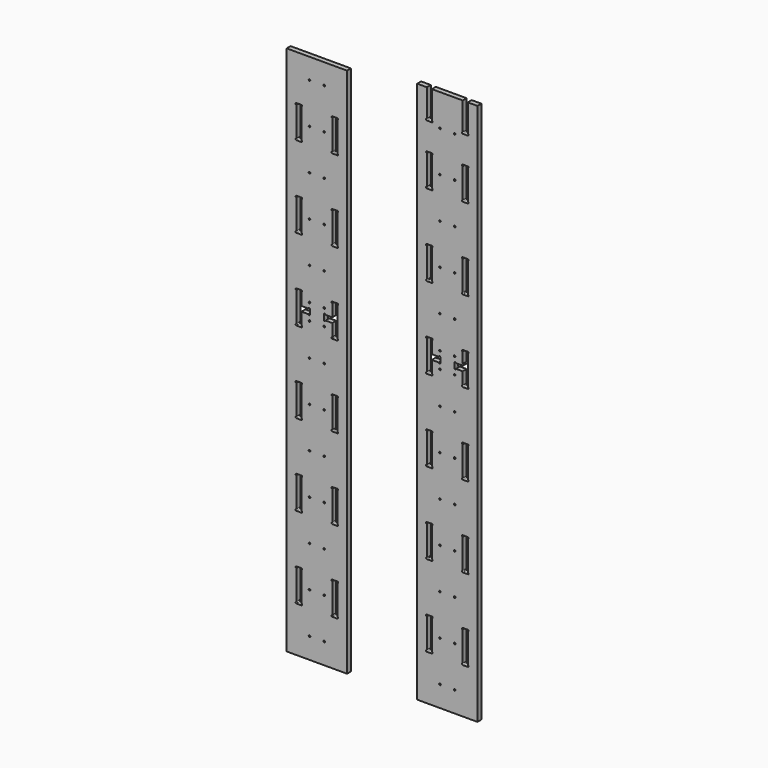
from build123d import *

# Parameters (mm, degrees)
F1_DEPTH = 18
F2_DEPTH = 18


# Not quite as in the source:
# - ends of sketch curves that miss each other by under 0.0002 mm in the source are joined


with BuildPart() as f1:
    # F0 (on Front) → F1 (new body)
    with BuildSketch(Plane.XZ):
        Polygon((-352.999778, -1175), (-352.999778, 777.505258), (-575.000001, 777.5052587556), (-575, -1175), align=None)
        with BuildLine():
            ThreePointArc((-491.003598, -1100.999773), (-493.1249183436, -1100.1210933436), (-494.003598, -1097.999773))
            ThreePointArc((-494.003598, -1097.999773), (-493.1249183436, -1095.8784526564), (-491.003598, -1094.999773))
            ThreePointArc((-491.003598, -1094.999773), (-488.8822776564, -1095.8784526564), (-488.003598, -1097.999773))
            ThreePointArc((-488.003598, -1097.999773), (-488.8822776564, -1100.1210933436), (-491.003598, -1100.999773))
        make_face(mode=Mode.SUBTRACT)
        with BuildLine():
            Line((-520.753598, -1008.249833), (-539.253616, -1008.249833))
            ThreePointArc((-539.253616, -1008.249833), (-542.263616, -1005.239833), (-539.253616, -1002.229833))
            Line((-539.253616, -1002.229833), (-539.253616, -893.769713))
            ThreePointArc((-539.253616, -893.769713), (-542.263616, -890.759713), (-539.253616, -887.749713))
            Line((-539.253616, -887.749713), (-520.753598, -887.749713))
            ThreePointArc((-520.753598, -887.749713), (-517.743598, -890.759713), (-520.753598, -893.769713))
            Line((-520.753598, -893.769713), (-520.753598, -1002.229833))
            ThreePointArc((-520.753598, -1002.229833), (-517.743598, -1005.239833), (-520.753598, -1008.249833))
        make_face(mode=Mode.SUBTRACT)
        with BuildLine():
            ThreePointArc((-491.003598, -950.999773), (-493.1249183436, -950.1210933436), (-494.003598, -947.999773))
            ThreePointArc((-494.003598, -947.999773), (-493.1249183436, -945.8784526564), (-491.003598, -944.999773))
            ThreePointArc((-491.003598, -944.999773), (-488.8822776564, -945.8784526564), (-488.003598, -947.999773))
            ThreePointArc((-488.003598, -947.999773), (-488.8822776564, -950.1210933436), (-491.003598, -950.999773))
        make_face(mode=Mode.SUBTRACT)
        with BuildLine():
            ThreePointArc((-437.003484, -1100.999773), (-439.1248043436, -1100.1210933436), (-440.003484, -1097.999773))
            ThreePointArc((-440.003484, -1097.999773), (-439.1248043436, -1095.8784526564), (-437.003484, -1094.999773))
            ThreePointArc((-437.003484, -1094.999773), (-434.8821636564, -1095.8784526564), (-434.003484, -1097.999773))
            ThreePointArc((-434.003484, -1097.999773), (-434.8821636564, -1100.1210933436), (-437.003484, -1100.999773))
        make_face(mode=Mode.SUBTRACT)
        with BuildLine():
            ThreePointArc((-437.003484, -950.999773), (-439.1248043436, -950.1210933436), (-440.003484, -947.999773))
            ThreePointArc((-440.003484, -947.999773), (-439.1248043436, -945.8784526564), (-437.003484, -944.999773))
            ThreePointArc((-437.003484, -944.999773), (-434.8821636564, -945.8784526564), (-434.003484, -947.999773))
            ThreePointArc((-434.003484, -947.999773), (-434.8821636564, -950.1210933436), (-437.003484, -950.999773))
        make_face(mode=Mode.SUBTRACT)
        with BuildLine():
            Line((-388.753466, -893.769713), (-388.753466, -1002.229833))
            ThreePointArc((-388.753466, -1002.229833), (-385.743466, -1005.239833), (-388.753466, -1008.249833))
            Line((-388.753466, -1008.249833), (-407.253484, -1008.249833))
            ThreePointArc((-407.253484, -1008.249833), (-410.263484, -1005.239833), (-407.253484, -1002.229833))
            Line((-407.253484, -1002.229833), (-407.253484, -893.769713))
            ThreePointArc((-407.253484, -893.769713), (-410.263484, -890.759713), (-407.253484, -887.749713))
            Line((-407.253484, -887.749713), (-388.753466, -887.749713))
            ThreePointArc((-388.753466, -887.749713), (-385.743466, -890.759713), (-388.753466, -893.769713))
        make_face(mode=Mode.SUBTRACT)
        with BuildLine():
            ThreePointArc((-491.003598, -800.999773), (-493.1249183436, -800.1210933436), (-494.003598, -797.999773))
            ThreePointArc((-494.003598, -797.999773), (-493.1249183436, -795.8784526564), (-491.003598, -794.999773))
            ThreePointArc((-491.003598, -794.999773), (-488.8822776564, -795.8784526564), (-488.003598, -797.999773))
            ThreePointArc((-488.003598, -797.999773), (-488.8822776564, -800.1210933436), (-491.003598, -800.999773))
        make_face(mode=Mode.SUBTRACT)
        with BuildLine():
            Line((-520.749918, -593.769409), (-520.749918, -702.229597))
            ThreePointArc((-520.749918, -702.229597), (-517.739918, -705.239597), (-520.749918, -708.249597))
            Line((-520.749918, -708.249597), (-539.249936, -708.249597))
            ThreePointArc((-539.249936, -708.249597), (-542.259936, -705.239597), (-539.249936, -702.229597))
            Line((-539.249936, -702.229597), (-539.249936, -593.769409))
            ThreePointArc((-539.249936, -593.769409), (-542.259936, -590.759409), (-539.249936, -587.749409))
            Line((-539.249936, -587.749409), (-520.749918, -587.749409))
            ThreePointArc((-520.749918, -587.749409), (-517.739918, -590.759409), (-520.749918, -593.769409))
        make_face(mode=Mode.SUBTRACT)
        with BuildLine():
            ThreePointArc((-491.003598, -650.999773), (-493.1249183436, -650.1210933436), (-494.003598, -647.999773))
            ThreePointArc((-494.003598, -647.999773), (-493.1249183436, -645.8784526564), (-491.003598, -644.999773))
            ThreePointArc((-491.003598, -644.999773), (-488.8822776564, -645.8784526564), (-488.003598, -647.999773))
            ThreePointArc((-488.003598, -647.999773), (-488.8822776564, -650.1210933436), (-491.003598, -650.999773))
        make_face(mode=Mode.SUBTRACT)
        with BuildLine():
            ThreePointArc((-437.003484, -800.999773), (-439.1248043436, -800.1210933436), (-440.003484, -797.999773))
            ThreePointArc((-440.003484, -797.999773), (-439.1248043436, -795.8784526564), (-437.003484, -794.999773))
            ThreePointArc((-437.003484, -794.999773), (-434.8821636564, -795.8784526564), (-434.003484, -797.999773))
            ThreePointArc((-434.003484, -797.999773), (-434.8821636564, -800.1210933436), (-437.003484, -800.999773))
        make_face(mode=Mode.SUBTRACT)
        with BuildLine():
            ThreePointArc((-437.003484, -650.999773), (-439.1248043436, -650.1210933436), (-440.003484, -647.999773))
            ThreePointArc((-440.003484, -647.999773), (-439.1248043436, -645.8784526564), (-437.003484, -644.999773))
            ThreePointArc((-437.003484, -644.999773), (-434.8821636564, -645.8784526564), (-434.003484, -647.999773))
            ThreePointArc((-434.003484, -647.999773), (-434.8821636564, -650.1210933436), (-437.003484, -650.999773))
        make_face(mode=Mode.SUBTRACT)
        with BuildLine():
            Line((-388.749807, -593.768176), (-388.749807, -702.228296))
            ThreePointArc((-388.749807, -702.228296), (-385.739807, -705.238296), (-388.749807, -708.248296))
            Line((-388.749807, -708.248296), (-407.249825, -708.248296))
            ThreePointArc((-407.249825, -708.248296), (-410.259825, -705.238296), (-407.249825, -702.228296))
            Line((-407.249825, -702.228296), (-407.249825, -593.768176))
            ThreePointArc((-407.249825, -593.768176), (-410.259825, -590.758176), (-407.249825, -587.748176))
            Line((-407.249825, -587.748176), (-388.749807, -587.748176))
            ThreePointArc((-388.749807, -587.748176), (-385.739807, -590.758176), (-388.749807, -593.768176))
        make_face(mode=Mode.SUBTRACT)
        with BuildLine():
            ThreePointArc((-491.003598, -500.999773), (-493.1249183436, -500.1210933436), (-494.003598, -497.999773))
            ThreePointArc((-494.003598, -497.999773), (-493.1249183436, -495.8784526564), (-491.003598, -494.999773))
            ThreePointArc((-491.003598, -494.999773), (-488.8822776564, -495.8784526564), (-488.003598, -497.999773))
            ThreePointArc((-488.003598, -497.999773), (-488.8822776564, -500.1210933436), (-491.003598, -500.999773))
        make_face(mode=Mode.SUBTRACT)
        with BuildLine():
            Line((-520.749849, -293.766172), (-520.749849, -402.226361))
            ThreePointArc((-520.749849, -402.226361), (-517.739849, -405.236361), (-520.749849, -408.246361))
            Line((-520.749849, -408.246361), (-539.249867, -408.246361))
            ThreePointArc((-539.249867, -408.246361), (-542.259867, -405.236361), (-539.249867, -402.226361))
            Line((-539.249867, -402.226361), (-539.249867, -293.766172))
            ThreePointArc((-539.249867, -293.766172), (-542.259867, -290.756172), (-539.249867, -287.746172))
            Line((-539.249867, -287.746172), (-520.749849, -287.746172))
            ThreePointArc((-520.749849, -287.746172), (-517.739849, -290.756172), (-520.749849, -293.766172))
        make_face(mode=Mode.SUBTRACT)
        with BuildLine():
            ThreePointArc((-491.003598, -350.999773), (-493.1249183436, -350.1210933436), (-494.003598, -347.999773))
            ThreePointArc((-494.003598, -347.999773), (-493.1249183436, -345.8784526564), (-491.003598, -344.999773))
            ThreePointArc((-491.003598, -344.999773), (-488.8822776564, -345.8784526564), (-488.003598, -347.999773))
            ThreePointArc((-488.003598, -347.999773), (-488.8822776564, -350.1210933436), (-491.003598, -350.999773))
        make_face(mode=Mode.SUBTRACT)
        with BuildLine():
            ThreePointArc((-437.003484, -500.999773), (-439.1248043436, -500.1210933436), (-440.003484, -497.999773))
            ThreePointArc((-440.003484, -497.999773), (-439.1248043436, -495.8784526564), (-437.003484, -494.999773))
            ThreePointArc((-437.003484, -494.999773), (-434.8821636564, -495.8784526564), (-434.003484, -497.999773))
            ThreePointArc((-434.003484, -497.999773), (-434.8821636564, -500.1210933436), (-437.003484, -500.999773))
        make_face(mode=Mode.SUBTRACT)
        with BuildLine():
            ThreePointArc((-437.003484, -350.999773), (-439.1248043436, -350.1210933436), (-440.003484, -347.999773))
            ThreePointArc((-440.003484, -347.999773), (-439.1248043436, -345.8784526564), (-437.003484, -344.999773))
            ThreePointArc((-437.003484, -344.999773), (-434.8821636564, -345.8784526564), (-434.003484, -347.999773))
            ThreePointArc((-434.003484, -347.999773), (-434.8821636564, -350.1210933436), (-437.003484, -350.999773))
        make_face(mode=Mode.SUBTRACT)
        with BuildLine():
            Line((-407.249756, -402.225059), (-407.249756, -293.764939))
            ThreePointArc((-407.249756, -293.764939), (-410.259756, -290.754939), (-407.249756, -287.744939))
            Line((-407.249756, -287.744939), (-388.749738, -287.744939))
            ThreePointArc((-388.749738, -287.744939), (-385.739738, -290.754939), (-388.749738, -293.764939))
            Line((-388.749738, -293.764939), (-388.749738, -402.225059))
            ThreePointArc((-388.749738, -402.225059), (-385.739738, -405.235059), (-388.749738, -408.245059))
            Line((-388.749738, -408.245059), (-407.249756, -408.245059))
            ThreePointArc((-407.249756, -408.245059), (-410.259756, -405.235059), (-407.249756, -402.225059))
        make_face(mode=Mode.SUBTRACT)
        with BuildLine():
            ThreePointArc((-491.003598, -200.999773), (-493.1249183436, -200.1210933436), (-494.003598, -197.999773))
            ThreePointArc((-494.003598, -197.999773), (-493.1249183436, -195.8784526564), (-491.003598, -194.999773))
            ThreePointArc((-491.003598, -194.999773), (-488.8822776564, -195.8784526564), (-488.003598, -197.999773))
            ThreePointArc((-488.003598, -197.999773), (-488.8822776564, -200.1210933436), (-491.003598, -200.999773))
        make_face(mode=Mode.SUBTRACT)
        with BuildLine():
            ThreePointArc((-491.003598, -80.986601), (-493.1249183436, -80.1079213436), (-494.003598, -77.986601))
            ThreePointArc((-494.003598, -77.986601), (-493.1249183436, -75.8652806564), (-491.003598, -74.986601))
            ThreePointArc((-491.003598, -74.986601), (-488.8822776564, -75.8652806564), (-488.003598, -77.986601))
            ThreePointArc((-488.003598, -77.986601), (-488.8822776564, -80.1079213436), (-491.003598, -80.986601))
        make_face(mode=Mode.SUBTRACT)
        with BuildLine():
            Line((-520.749955, 6.236645), (-520.749974, -38.743178))
            Line((-520.749974, -38.743178), (-495.769943, -38.743178))
            ThreePointArc((-495.769943, -38.743178), (-492.759943, -35.733178), (-489.749943, -38.743178))
            Line((-489.749943, -38.743178), (-489.749943, -57.243196))
            ThreePointArc((-489.749943, -57.243196), (-492.759943, -60.253196), (-495.769943, -57.243196))
            Line((-495.769943, -57.243196), (-520.749974, -57.243196))
            Line((-520.749974, -57.243196), (-520.749955, -102.223475))
            ThreePointArc((-520.749955, -102.223475), (-517.739954, -105.233474), (-520.749953, -108.243475))
            Line((-520.749953, -108.243475), (-539.249971, -108.243475))
            ThreePointArc((-539.249971, -108.243475), (-542.259971, -105.233475), (-539.249971, -102.223475))
            Line((-539.249971, -102.223475), (-539.249971, 6.236645))
            ThreePointArc((-539.249971, 6.236645), (-542.259971, 9.246645), (-539.249971, 12.256645))
            Line((-539.249971, 12.256645), (-520.749953, 12.256645))
            ThreePointArc((-520.749953, 12.256645), (-517.739954, 9.246644), (-520.749955, 6.236645))
        make_face(mode=Mode.SUBTRACT)
        with BuildLine():
            ThreePointArc((-491.003598, -20.999773), (-493.1249183436, -20.1210933436), (-494.003598, -17.999773))
            ThreePointArc((-494.003598, -17.999773), (-493.1249183436, -15.8784526564), (-491.003598, -14.999773))
            ThreePointArc((-491.003598, -14.999773), (-488.8822776564, -15.8784526564), (-488.003598, -17.999773))
            ThreePointArc((-488.003598, -17.999773), (-488.8822776564, -20.1210933436), (-491.003598, -20.999773))
        make_face(mode=Mode.SUBTRACT)
        with BuildLine():
            ThreePointArc((-437.003484, -200.999773), (-439.1248043436, -200.1210933436), (-440.003484, -197.999773))
            ThreePointArc((-440.003484, -197.999773), (-439.1248043436, -195.8784526564), (-437.003484, -194.999773))
            ThreePointArc((-437.003484, -194.999773), (-434.8821636564, -195.8784526564), (-434.003484, -197.999773))
            ThreePointArc((-434.003484, -197.999773), (-434.8821636564, -200.1210933436), (-437.003484, -200.999773))
        make_face(mode=Mode.SUBTRACT)
        with BuildLine():
            ThreePointArc((-437.003484, -80.986601), (-439.1248043436, -80.1079213436), (-440.003484, -77.986601))
            ThreePointArc((-440.003484, -77.986601), (-439.1248043436, -75.8652806564), (-437.003484, -74.986601))
            ThreePointArc((-437.003484, -74.986601), (-434.8821636564, -75.8652806564), (-434.003484, -77.986601))
            ThreePointArc((-434.003484, -77.986601), (-434.8821636564, -80.1079213436), (-437.003484, -80.986601))
        make_face(mode=Mode.SUBTRACT)
        with BuildLine():
            ThreePointArc((-437.003484, -20.999773), (-439.1248043436, -20.1210933436), (-440.003484, -17.999773))
            ThreePointArc((-440.003484, -17.999773), (-439.1248043436, -15.8784526564), (-437.003484, -14.999773))
            ThreePointArc((-437.003484, -14.999773), (-434.8821636564, -15.8784526564), (-434.003484, -17.999773))
            ThreePointArc((-434.003484, -17.999773), (-434.8821636564, -20.1210933436), (-437.003484, -20.999773))
        make_face(mode=Mode.SUBTRACT)
        with BuildLine():
            Line((-388.749842, 6.235389), (-388.749842, -102.224782))
            ThreePointArc((-388.749842, -102.224782), (-385.739842, -105.234782), (-388.749842, -108.244782))
            Line((-388.749842, -108.244782), (-407.249855, -108.244782))
            ThreePointArc((-407.249855, -108.2447819994), (-410.2599159994, -105.2348425), (-407.249976, -102.2247820006))
            Line((-407.249976, -102.224782), (-407.250887, -57.243196))
            Line((-407.250887, -57.243196), (-432.230923, -57.243196))
            ThreePointArc((-432.230923, -57.243196), (-435.240923, -60.253196), (-438.250923, -57.243196))
            Line((-438.250923, -57.243196), (-438.250923, -38.743178))
            ThreePointArc((-438.250923, -38.743178), (-435.240923, -35.733178), (-432.230923, -38.743178))
            Line((-432.230923, -38.743178), (-407.250887, -38.743178))
            Line((-407.250887, -38.743178), (-407.249976, 6.235389))
            ThreePointArc((-407.249976, 6.2353890006), (-410.2599159994, 9.2454495), (-407.249855, 12.2553889994))
            Line((-407.249855, 12.255389), (-388.749842, 12.255389))
            ThreePointArc((-388.749842, 12.255389), (-385.739842, 9.245389), (-388.749842, 6.235389))
        make_face(mode=Mode.SUBTRACT)
        with BuildLine():
            ThreePointArc((-491.003598, 99.000227), (-493.1249183436, 99.8789066564), (-494.003598, 102.000227))
            ThreePointArc((-494.003598, 102.000227), (-493.1249183436, 104.1215473436), (-491.003598, 105.000227))
            ThreePointArc((-491.003598, 105.000227), (-488.8822776564, 104.1215473436), (-488.003598, 102.000227))
            ThreePointArc((-488.003598, 102.000227), (-488.8822776564, 99.8789066564), (-491.003598, 99.000227))
        make_face(mode=Mode.SUBTRACT)
        with BuildLine():
            Line((-520.749918, 306.234452), (-520.749918, 197.774263))
            ThreePointArc((-520.749918, 197.774263), (-517.739918, 194.764263), (-520.749918, 191.754263))
            Line((-520.749918, 191.754263), (-539.249936, 191.754263))
            ThreePointArc((-539.249936, 191.754263), (-542.259936, 194.764263), (-539.249936, 197.774263))
            Line((-539.249936, 197.774263), (-539.249936, 306.234452))
            ThreePointArc((-539.249936, 306.234452), (-542.259936, 309.244452), (-539.249936, 312.254452))
            Line((-539.249936, 312.254452), (-520.749918, 312.254452))
            ThreePointArc((-520.749918, 312.254452), (-517.739918, 309.244452), (-520.749918, 306.234452))
        make_face(mode=Mode.SUBTRACT)
        with BuildLine():
            ThreePointArc((-491.003598, 249.000227), (-493.1249183436, 249.8789066564), (-494.003598, 252.000227))
            ThreePointArc((-494.003598, 252.000227), (-493.1249183436, 254.1215473436), (-491.003598, 255.000227))
            ThreePointArc((-491.003598, 255.000227), (-488.8822776564, 254.1215473436), (-488.003598, 252.000227))
            ThreePointArc((-488.003598, 252.000227), (-488.8822776564, 249.8789066564), (-491.003598, 249.000227))
        make_face(mode=Mode.SUBTRACT)
        with BuildLine():
            ThreePointArc((-437.003484, 99.000227), (-439.1248043436, 99.8789066564), (-440.003484, 102.000227))
            ThreePointArc((-440.003484, 102.000227), (-439.1248043436, 104.1215473436), (-437.003484, 105.000227))
            ThreePointArc((-437.003484, 105.000227), (-434.8821636564, 104.1215473436), (-434.003484, 102.000227))
            ThreePointArc((-434.003484, 102.000227), (-434.8821636564, 99.8789066564), (-437.003484, 99.000227))
        make_face(mode=Mode.SUBTRACT)
        with BuildLine():
            ThreePointArc((-437.003484, 249.000227), (-439.1248043436, 249.8789066564), (-440.003484, 252.000227))
            ThreePointArc((-440.003484, 252.000227), (-439.1248043436, 254.1215473436), (-437.003484, 255.000227))
            ThreePointArc((-437.003484, 255.000227), (-434.8821636564, 254.1215473436), (-434.003484, 252.000227))
            ThreePointArc((-434.003484, 252.000227), (-434.8821636564, 249.8789066564), (-437.003484, 249.000227))
        make_face(mode=Mode.SUBTRACT)
        with BuildLine():
            Line((-407.249825, 197.775565), (-407.249825, 306.235685))
            ThreePointArc((-407.249825, 306.235685), (-410.259825, 309.245685), (-407.249825, 312.255685))
            Line((-407.249825, 312.255685), (-388.749807, 312.255685))
            ThreePointArc((-388.749807, 312.255685), (-385.739807, 309.245685), (-388.749807, 306.235685))
            Line((-388.749807, 306.235685), (-388.749807, 197.775565))
            ThreePointArc((-388.749807, 197.775565), (-385.739807, 194.765565), (-388.749807, 191.755565))
            Line((-388.749807, 191.755565), (-407.249825, 191.755565))
            ThreePointArc((-407.249825, 191.755565), (-410.259825, 194.765565), (-407.249825, 197.775565))
        make_face(mode=Mode.SUBTRACT)
        with BuildLine():
            ThreePointArc((-491.003598, 399.000227), (-493.1249183436, 399.8789066564), (-494.003598, 402.000227))
            ThreePointArc((-494.003598, 402.000227), (-493.1249183436, 404.1215473436), (-491.003598, 405.000227))
            ThreePointArc((-491.003598, 405.000227), (-488.8822776564, 404.1215473436), (-488.003598, 402.000227))
            ThreePointArc((-488.003598, 402.000227), (-488.8822776564, 399.8789066564), (-491.003598, 399.000227))
        make_face(mode=Mode.SUBTRACT)
        with BuildLine():
            Line((-539.249936, 497.774554), (-539.249936, 606.234743))
            ThreePointArc((-539.249936, 606.234743), (-542.259936, 609.244743), (-539.249936, 612.254743))
            Line((-539.249936, 612.254743), (-520.749918, 612.254743))
            ThreePointArc((-520.749918, 612.254743), (-517.739918, 609.244743), (-520.749918, 606.234743))
            Line((-520.749918, 606.234743), (-520.749918, 497.774554))
            ThreePointArc((-520.749918, 497.774554), (-517.739918, 494.764554), (-520.749918, 491.754554))
            Line((-520.749918, 491.754554), (-539.249936, 491.754554))
            ThreePointArc((-539.249936, 491.754554), (-542.259936, 494.764554), (-539.249936, 497.774554))
        make_face(mode=Mode.SUBTRACT)
        with BuildLine():
            ThreePointArc((-491.003598, 549.000227), (-493.1249183436, 549.8789066564), (-494.003598, 552.000227))
            ThreePointArc((-494.003598, 552.000227), (-493.1249183436, 554.1215473436), (-491.003598, 555.000227))
            ThreePointArc((-491.003598, 555.000227), (-488.8822776564, 554.1215473436), (-488.003598, 552.000227))
            ThreePointArc((-488.003598, 552.000227), (-488.8822776564, 549.8789066564), (-491.003598, 549.000227))
        make_face(mode=Mode.SUBTRACT)
        with BuildLine():
            ThreePointArc((-437.003484, 399.000227), (-439.1248043436, 399.8789066564), (-440.003484, 402.000227))
            ThreePointArc((-440.003484, 402.000227), (-439.1248043436, 404.1215473436), (-437.003484, 405.000227))
            ThreePointArc((-437.003484, 405.000227), (-434.8821636564, 404.1215473436), (-434.003484, 402.000227))
            ThreePointArc((-434.003484, 402.000227), (-434.8821636564, 399.8789066564), (-437.003484, 399.000227))
        make_face(mode=Mode.SUBTRACT)
        with BuildLine():
            ThreePointArc((-437.003484, 549.000227), (-439.1248043436, 549.8789066564), (-440.003484, 552.000227))
            ThreePointArc((-440.003484, 552.000227), (-439.1248043436, 554.1215473436), (-437.003484, 555.000227))
            ThreePointArc((-437.003484, 555.000227), (-434.8821636564, 554.1215473436), (-434.003484, 552.000227))
            ThreePointArc((-434.003484, 552.000227), (-434.8821636564, 549.8789066564), (-437.003484, 549.000227))
        make_face(mode=Mode.SUBTRACT)
        with BuildLine():
            Line((-388.749807, 606.235976), (-388.749807, 497.775856))
            ThreePointArc((-388.749807, 497.775856), (-385.739807, 494.765856), (-388.749807, 491.755856))
            Line((-388.749807, 491.755856), (-407.249825, 491.755856))
            ThreePointArc((-407.249825, 491.755856), (-410.259825, 494.765856), (-407.249825, 497.775856))
            Line((-407.249825, 497.775856), (-407.249825, 606.235976))
            ThreePointArc((-407.249825, 606.235976), (-410.259825, 609.245976), (-407.249825, 612.255976))
            Line((-407.249825, 612.255976), (-388.749807, 612.255976))
            ThreePointArc((-388.749807, 612.255976), (-385.739807, 609.245976), (-388.749807, 606.235976))
        make_face(mode=Mode.SUBTRACT)
        Polygon((-506.973918, 655.086016), (-522.336584, 655.086016), (-522.336584, 672.56035), (-506.973918, 672.56035), (-506.541339, 672.557371), (-506.111272, 672.53204), (-505.684535, 672.484696), (-505.261944, 672.415683), (-504.844315, 672.325341), (-504.432466, 672.214014), (-504.027214, 672.082041), (-503.629376, 671.929766), (-503.239768, 671.75753), (-502.859207, 671.565675), (-502.488511, 671.354543), (-502.128496, 671.124475), (-501.779978, 670.875813), (-501.443776, 670.608899), (-501.120706, 670.324075), (-500.811584, 670.021683), (-500.5137, 669.714114), (-500.232763, 669.39305), (-499.969092, 669.059272), (-499.723011, 668.713558), (-499.49484, 668.356688), (-499.284901, 667.989441), (-499.093514, 667.612596), (-498.921001, 667.226933), (-498.767683, 666.833231), (-498.633882, 666.432269), (-498.519919, 666.024827), (-498.426115, 665.611683), (-498.352792, 665.193618), (-498.30027, 664.77141), (-498.268872, 664.345838), (-498.258918, 663.917683), (-498.256319, 663.478817), (-498.276304, 663.042145), (-498.318539, 662.608495), (-498.382694, 662.178693), (-498.468436, 661.753568), (-498.575435, 661.333945), (-498.703359, 660.920652), (-498.851876, 660.514516), (-499.020655, 660.116365), (-499.209363, 659.727025), (-499.417671, 659.347324), (-499.645246, 658.978089), (-499.891756, 658.620147), (-500.15687, 658.274325), (-500.440257, 657.94145), (-500.741584, 657.62235), (-501.056696, 657.32124), (-501.385493, 657.037626), (-501.727169, 656.771834), (-502.080918, 656.524188), (-502.445932, 656.295013), (-502.821404, 656.084633), (-503.20653, 655.893373), (-503.600501, 655.721558), (-504.002511, 655.569512), (-504.411753, 655.437561), (-504.827422, 655.326029), (-505.248709, 655.23524), (-505.674809, 655.16552), (-506.104915, 655.117193), (-506.53822, 655.090583), align=None, mode=Mode.SUBTRACT)
        Polygon((-475.769852, 637.107772), (-476.131918, 637.10535), (-476.499301, 637.102372), (-476.8659, 637.108707), (-477.231546, 637.124288), (-477.596071, 637.14905), (-477.959305, 637.182925), (-478.32108, 637.225848), (-478.681228, 637.277753), (-479.039579, 637.338574), (-479.395965, 637.408243), (-479.750216, 637.486695), (-480.102165, 637.573864), (-480.451642, 637.669684), (-480.798479, 637.774087), (-481.142506, 637.887009), (-481.483556, 638.008382), (-481.821459, 638.138141), (-482.156047, 638.27622), (-482.48715, 638.422551), (-482.814601, 638.577069), (-483.138229, 638.739708), (-483.457868, 638.910402), (-483.773347, 639.089083), (-484.084498, 639.275687), (-484.391152, 639.470147), (-484.693141, 639.672395), (-484.990295, 639.882368), (-485.282446, 640.099997), (-485.569426, 640.325217), (-485.851065, 640.557962), (-486.127195, 640.798166), (-486.397646, 641.045761), (-486.662251, 641.300683), (-486.968379, 641.633429), (-487.26546, 641.973094), (-487.553417, 642.319472), (-487.832171, 642.672359), (-488.101646, 643.031551), (-488.361764, 643.396843), (-488.612446, 643.76803), (-488.853615, 644.144907), (-489.085194, 644.52727), (-489.307104, 644.914914), (-489.519267, 645.307635), (-489.721606, 645.705228), (-489.914044, 646.107488), (-490.096502, 646.51421), (-490.268902, 646.925191), (-490.431168, 647.340225), (-490.58322, 647.759107), (-490.724982, 648.181633), (-490.856375, 648.607599), (-490.977322, 649.0368), (-491.087746, 649.46903), (-491.187567, 649.904086), (-491.27671, 650.341762), (-491.355095, 650.781855), (-491.422645, 651.224159), (-491.479282, 651.66847), (-491.524929, 652.114583), (-491.559507, 652.562293), (-491.58294, 653.011396), (-491.595149, 653.461688), (-491.596056, 653.912963), (-491.585584, 654.365016), (-491.599646, 654.855997), (-491.601202, 655.346163), (-491.590337, 655.835287), (-491.567136, 656.323143), (-491.531686, 656.809504), (-491.484071, 657.294142), (-491.424376, 657.776831), (-491.352688, 658.257344), (-491.269092, 658.735455), (-491.173673, 659.210935), (-491.066517, 659.68356), (-490.947709, 660.1531), (-490.817335, 660.619331), (-490.675479, 661.082024), (-490.522228, 661.540953), (-490.357668, 661.995891), (-490.181882, 662.446612), (-489.994957, 662.892888), (-489.796979, 663.334492), (-489.588032, 663.771198), (-489.368203, 664.202779), (-489.137576, 664.629007), (-488.896237, 665.049657), (-488.644272, 665.464501), (-488.381765, 665.873312), (-488.108804, 666.275863), (-487.825472, 666.671928), (-487.531855, 667.06128), (-487.228039, 667.443692), (-486.91411, 667.818936), (-486.590152, 668.186787), (-486.256251, 668.547016), (-486.006221, 668.801356), (-485.750182, 669.048515), (-485.488307, 669.288422), (-485.220766, 669.521005), (-484.94773, 669.746194), (-484.669372, 669.963916), (-484.385861, 670.174102), (-484.097371, 670.376678), (-483.804071, 670.571574), (-483.506133, 670.758718), (-483.203729, 670.93804), (-482.89703, 671.109467), (-482.586207, 671.272929), (-482.271432, 671.428354), (-481.952875, 671.575671), (-481.630709, 671.714808), (-481.305104, 671.845694), (-480.976233, 671.968258), (-480.644265, 672.082428), (-480.309373, 672.188133), (-479.971727, 672.285301), (-479.6315, 672.373862), (-479.288862, 672.453744), (-478.943985, 672.524876), (-478.59704, 672.587185), (-478.248199, 672.640602), (-477.897632, 672.685054), (-477.545512, 672.72047), (-477.192009, 672.746779), (-476.837295, 672.76391), (-476.48154, 672.77179), (-476.124918, 672.77035), (-475.76245, 672.767135), (-475.400977, 672.754479), (-475.040671, 672.732456), (-474.681705, 672.701138), (-474.324254, 672.6606), (-473.96849, 672.610917), (-473.614588, 672.552161), (-473.26272, 672.484407), (-472.91306, 672.407729), (-472.565781, 672.3222), (-472.221057, 672.227895), (-471.879062, 672.124887), (-471.539969, 672.01325), (-471.203951, 671.893059), (-470.871181, 671.764387), (-470.541834, 671.627308), (-470.216083, 671.481896), (-469.894101, 671.328225), (-469.576061, 671.166369), (-469.262138, 670.996401), (-468.952504, 670.818396), (-468.647333, 670.632428), (-468.346798, 670.43857), (-468.051074, 670.236897), (-467.760333, 670.027481), (-467.474748, 669.810398), (-467.194494, 669.585722), (-466.919744, 669.353525), (-466.650671, 669.113882), (-466.387449, 668.866867), (-466.130251, 668.612554), (-465.879251, 668.351016), (-465.555343, 667.992679), (-465.241237, 667.627003), (-464.937012, 667.25421), (-464.642748, 666.874522), (-464.358527, 666.48816), (-464.084428, 666.095347), (-463.820531, 665.696303), (-463.566918, 665.291251), (-463.323667, 664.880412), (-463.090861, 664.464008), (-462.868578, 664.042261), (-462.656899, 663.615393), (-462.455905, 663.183625), (-462.265676, 662.74718), (-462.086292, 662.306278), (-461.917834, 661.861141), (-461.760382, 661.411992), (-461.614015, 660.959052), (-461.478816, 660.502543), (-461.354863, 660.042686), (-461.242237, 659.579704), (-461.141019, 659.113817), (-461.051288, 658.645249), (-460.973126, 658.174219), (-460.906612, 657.700951), (-460.851827, 657.225666), (-460.808851, 656.748586), (-460.777764, 656.269932), (-460.758647, 655.789927), (-460.75158, 655.308791), (-460.756643, 654.826747), (-460.773918, 654.344016), (-460.766542, 653.893542), (-460.770611, 653.443945), (-460.786045, 652.995432), (-460.812764, 652.548211), (-460.850687, 652.102489), (-460.899733, 651.658472), (-460.959823, 651.216369), (-461.030876, 650.776386), (-461.112812, 650.338731), (-461.20555, 649.903611), (-461.30901, 649.471232), (-461.423113, 649.041803), (-461.547777, 648.615531), (-461.682922, 648.192622), (-461.828468, 647.773284), (-461.984334, 647.357725), (-462.150441, 646.94615), (-462.326708, 646.538768), (-462.513054, 646.135786), (-462.709399, 645.737411), (-462.915664, 645.343851), (-463.131767, 644.955311), (-463.357628, 644.572001), (-463.593168, 644.194126), (-463.838305, 643.821894), (-464.092959, 643.455512), (-464.35705, 643.095188), (-464.630498, 642.741129), (-464.913223, 642.393542), (-465.205143, 642.052633), (-465.506179, 641.718611), (-465.816251, 641.391683), (-466.073419, 641.136871), (-466.336438, 640.889169), (-466.605143, 640.648646), (-466.879371, 640.41537), (-467.158957, 640.18941), (-467.443735, 639.970835), (-467.733543, 639.759714), (-468.028214, 639.556115), (-468.327586, 639.360108), (-468.631492, 639.171761), (-468.939769, 638.991142), (-469.252253, 638.818322), (-469.568778, 638.653367), (-469.88918, 638.496348), (-470.213296, 638.347333), (-470.540959, 638.206391), (-470.872006, 638.073591), (-471.206273, 637.949001), (-471.543594, 637.83269), (-471.883806, 637.724727), (-472.226744, 637.62518), (-472.572243, 637.53412), (-472.920138, 637.451613), (-473.270266, 637.37773), (-473.622462, 637.312538), (-473.976562, 637.256108), (-474.3324, 637.208506), (-474.689813, 637.169803), (-475.048635, 637.140067), (-475.408703, 637.119367), align=None, mode=Mode.SUBTRACT)
        with BuildLine():
            ThreePointArc((-491.003598, 699.000227), (-493.1249183436, 699.8789066564), (-494.003598, 702.000227))
            ThreePointArc((-494.003598, 702.000227), (-493.1249183436, 704.1215473436), (-491.003598, 705.000227))
            ThreePointArc((-491.003598, 705.000227), (-488.8822776564, 704.1215473436), (-488.003598, 702.000227))
            ThreePointArc((-488.003598, 702.000227), (-488.8822776564, 699.8789066564), (-491.003598, 699.000227))
        make_face(mode=Mode.SUBTRACT)
        Polygon((-437.055185, 637.107772), (-437.417251, 637.10535), (-437.784634, 637.102372), (-438.151233, 637.108707), (-438.516879, 637.124288), (-438.881404, 637.14905), (-439.244638, 637.182925), (-439.606414, 637.225848), (-439.966561, 637.277753), (-440.324912, 637.338574), (-440.681298, 637.408243), (-441.03555, 637.486695), (-441.387498, 637.573864), (-441.736975, 637.669684), (-442.083812, 637.774087), (-442.42784, 637.887009), (-442.768889, 638.008382), (-443.106793, 638.138141), (-443.44138, 638.27622), (-443.772484, 638.422551), (-444.099934, 638.577069), (-444.423563, 638.739708), (-444.743201, 638.910402), (-445.05868, 639.089083), (-445.369831, 639.275687), (-445.676485, 639.470147), (-445.978474, 639.672395), (-446.275628, 639.882368), (-446.56778, 640.099997), (-446.854759, 640.325217), (-447.136398, 640.557962), (-447.412528, 640.798166), (-447.682979, 641.045761), (-447.947584, 641.300683), (-448.253712, 641.633429), (-448.550793, 641.973094), (-448.83875, 642.319472), (-449.117505, 642.672359), (-449.38698, 643.031551), (-449.647097, 643.396843), (-449.89778, 643.76803), (-450.138949, 644.144907), (-450.370527, 644.52727), (-450.592437, 644.914914), (-450.8046, 645.307635), (-451.00694, 645.705228), (-451.199377, 646.107488), (-451.381835, 646.51421), (-451.554235, 646.925191), (-451.716501, 647.340225), (-451.868553, 647.759107), (-452.010315, 648.181633), (-452.141709, 648.607599), (-452.262656, 649.0368), (-452.373079, 649.46903), (-452.472901, 649.904086), (-452.562043, 650.341762), (-452.640428, 650.781855), (-452.707978, 651.224159), (-452.764615, 651.66847), (-452.810262, 652.114583), (-452.844841, 652.562293), (-452.868273, 653.011396), (-452.880482, 653.461688), (-452.881389, 653.912963), (-452.870918, 654.365016), (-452.88498, 654.855997), (-452.886535, 655.346163), (-452.87567, 655.835287), (-452.85247, 656.323143), (-452.817019, 656.809504), (-452.769404, 657.294142), (-452.70971, 657.776831), (-452.638022, 658.257344), (-452.554426, 658.735455), (-452.459007, 659.210935), (-452.351851, 659.68356), (-452.233043, 660.1531), (-452.102668, 660.619331), (-451.960813, 661.082024), (-451.807562, 661.540953), (-451.643001, 661.995891), (-451.467215, 662.446612), (-451.280291, 662.892888), (-451.082312, 663.334492), (-450.873365, 663.771198), (-450.653536, 664.202779), (-450.422909, 664.629007), (-450.18157, 665.049657), (-449.929605, 665.464501), (-449.667099, 665.873312), (-449.394137, 666.275863), (-449.110805, 666.671928), (-448.817188, 667.06128), (-448.513373, 667.443692), (-448.199443, 667.818936), (-447.875485, 668.186787), (-447.541584, 668.547016), (-447.291554, 668.801356), (-447.035516, 669.048515), (-446.77364, 669.288422), (-446.506099, 669.521005), (-446.233064, 669.746194), (-445.954705, 669.963916), (-445.671195, 670.174102), (-445.382704, 670.376678), (-445.089404, 670.571574), (-444.791467, 670.758718), (-444.489063, 670.93804), (-444.182363, 671.109467), (-443.871541, 671.272929), (-443.556765, 671.428354), (-443.238209, 671.575671), (-442.916043, 671.714808), (-442.590438, 671.845694), (-442.261566, 671.968258), (-441.929598, 672.082428), (-441.594706, 672.188133), (-441.257061, 672.285301), (-440.916833, 672.373862), (-440.574196, 672.453744), (-440.229319, 672.524876), (-439.882374, 672.587185), (-439.533532, 672.640602), (-439.182966, 672.685054), (-438.830845, 672.72047), (-438.477342, 672.746779), (-438.122628, 672.76391), (-437.766874, 672.77179), (-437.410251, 672.77035), (-437.047784, 672.767135), (-436.68631, 672.754479), (-436.326004, 672.732456), (-435.967039, 672.701138), (-435.609587, 672.6606), (-435.253824, 672.610917), (-434.899921, 672.552161), (-434.548053, 672.484407), (-434.198393, 672.407729), (-433.851114, 672.3222), (-433.506391, 672.227895), (-433.164395, 672.124887), (-432.825302, 672.01325), (-432.489284, 671.893059), (-432.156515, 671.764387), (-431.827168, 671.627308), (-431.501416, 671.481896), (-431.179434, 671.328225), (-430.861394, 671.166369), (-430.547471, 670.996401), (-430.237837, 670.818396), (-429.932666, 670.632428), (-429.632132, 670.43857), (-429.336407, 670.236897), (-429.045666, 670.027481), (-428.760082, 669.810398), (-428.479828, 669.585722), (-428.205078, 669.353525), (-427.936005, 669.113882), (-427.672783, 668.866867), (-427.415585, 668.612554), (-427.164584, 668.351016), (-426.840677, 667.992679), (-426.52657, 667.627003), (-426.222345, 667.25421), (-425.928082, 666.874522), (-425.64386, 666.48816), (-425.369761, 666.095347), (-425.105864, 665.696303), (-424.852251, 665.291251), (-424.609001, 664.880412), (-424.376194, 664.464008), (-424.153911, 664.042261), (-423.942233, 663.615393), (-423.741239, 663.183625), (-423.55101, 662.74718), (-423.371626, 662.306278), (-423.203168, 661.861141), (-423.045715, 661.411992), (-422.899349, 660.959052), (-422.764149, 660.502543), (-422.640196, 660.042686), (-422.52757, 659.579704), (-422.426352, 659.113817), (-422.336622, 658.645249), (-422.258459, 658.174219), (-422.191945, 657.700951), (-422.13716, 657.225666), (-422.094184, 656.748586), (-422.063097, 656.269932), (-422.04398, 655.789927), (-422.036913, 655.308791), (-422.041977, 654.826747), (-422.059251, 654.344016), (-422.051875, 653.893542), (-422.055945, 653.443945), (-422.071379, 652.995432), (-422.098097, 652.548211), (-422.13602, 652.102489), (-422.185066, 651.658472), (-422.245156, 651.216369), (-422.316209, 650.776386), (-422.398145, 650.338731), (-422.490883, 649.903611), (-422.594344, 649.471232), (-422.708446, 649.041803), (-422.83311, 648.615531), (-422.968255, 648.192622), (-423.113801, 647.773284), (-423.269668, 647.357725), (-423.435774, 646.94615), (-423.612041, 646.538768), (-423.798387, 646.135786), (-423.994733, 645.737411), (-424.200997, 645.343851), (-424.4171, 644.955311), (-424.642961, 644.572001), (-424.878501, 644.194126), (-425.123638, 643.821894), (-425.378292, 643.455512), (-425.642384, 643.095188), (-425.915832, 642.741129), (-426.198556, 642.393542), (-426.490476, 642.052633), (-426.791513, 641.718611), (-427.101584, 641.391683), (-427.358752, 641.136871), (-427.621771, 640.889169), (-427.890477, 640.648646), (-428.164705, 640.41537), (-428.44429, 640.18941), (-428.729069, 639.970835), (-429.018876, 639.759714), (-429.313548, 639.556115), (-429.612919, 639.360108), (-429.916825, 639.171761), (-430.225103, 638.991142), (-430.537586, 638.818322), (-430.854111, 638.653367), (-431.174514, 638.496348), (-431.498629, 638.347333), (-431.826293, 638.206391), (-432.15734, 638.073591), (-432.491606, 637.949001), (-432.828928, 637.83269), (-433.16914, 637.724727), (-433.512077, 637.62518), (-433.857576, 637.53412), (-434.205472, 637.451613), (-434.5556, 637.37773), (-434.907796, 637.312538), (-435.261895, 637.256108), (-435.617733, 637.208506), (-435.975146, 637.169803), (-436.333969, 637.140067), (-436.694037, 637.119367), align=None, mode=Mode.SUBTRACT)
        with BuildLine():
            ThreePointArc((-437.003484, 699.000227), (-439.1248043436, 699.8789066564), (-440.003484, 702.000227))
            ThreePointArc((-440.003484, 702.000227), (-439.1248043436, 704.1215473436), (-437.003484, 705.000227))
            ThreePointArc((-437.003484, 705.000227), (-434.8821636564, 704.1215473436), (-434.003484, 702.000227))
            ThreePointArc((-434.003484, 702.000227), (-434.8821636564, 699.8789066564), (-437.003484, 699.000227))
        make_face(mode=Mode.SUBTRACT)
        Polygon((-522.336584, 672.56035), (-522.336584, 655.086016), (-506.973918, 655.086016), (-506.53822, 655.090583), (-506.104915, 655.117193), (-505.674809, 655.16552), (-505.248709, 655.23524), (-504.827422, 655.326029), (-504.411753, 655.437561), (-504.002511, 655.569512), (-503.600501, 655.721558), (-503.20653, 655.893373), (-502.821404, 656.084633), (-502.445932, 656.295013), (-502.080918, 656.524188), (-501.727169, 656.771834), (-501.385493, 657.037626), (-501.056696, 657.32124), (-500.741584, 657.62235), (-500.440257, 657.94145), (-500.15687, 658.274325), (-499.891756, 658.620147), (-499.645246, 658.978089), (-499.417671, 659.347324), (-499.209363, 659.727025), (-499.020655, 660.116365), (-498.851876, 660.514516), (-498.703359, 660.920652), (-498.575435, 661.333945), (-498.468436, 661.753568), (-498.382694, 662.178693), (-498.318539, 662.608495), (-498.276304, 663.042145), (-498.256319, 663.478817), (-498.258918, 663.917683), (-498.268872, 664.345838), (-498.30027, 664.77141), (-498.352792, 665.193618), (-498.426115, 665.611683), (-498.519919, 666.024827), (-498.633882, 666.432269), (-498.767683, 666.833231), (-498.921001, 667.226933), (-499.093514, 667.612596), (-499.284901, 667.989441), (-499.49484, 668.356688), (-499.723011, 668.713558), (-499.969092, 669.059272), (-500.232763, 669.39305), (-500.5137, 669.714114), (-500.811584, 670.021683), (-501.120706, 670.324075), (-501.443776, 670.608899), (-501.779978, 670.875813), (-502.128496, 671.124475), (-502.488511, 671.354543), (-502.859207, 671.565675), (-503.239768, 671.75753), (-503.629376, 671.929766), (-504.027214, 672.082041), (-504.432466, 672.214014), (-504.844315, 672.325341), (-505.261944, 672.415683), (-505.684535, 672.484696), (-506.111272, 672.53204), (-506.541339, 672.557371), (-506.973918, 672.56035), align=None)
        Polygon((-476.499301, 637.102372), (-476.131918, 637.10535), (-475.769852, 637.107772), (-475.408703, 637.119367), (-475.048635, 637.140067), (-474.689813, 637.169803), (-474.3324, 637.208506), (-473.976562, 637.256108), (-473.622462, 637.312538), (-473.270266, 637.37773), (-472.920138, 637.451613), (-472.572243, 637.53412), (-472.226744, 637.62518), (-471.883806, 637.724727), (-471.543594, 637.83269), (-471.206273, 637.949001), (-470.872006, 638.073591), (-470.540959, 638.206391), (-470.213296, 638.347333), (-469.88918, 638.496348), (-469.568778, 638.653367), (-469.252253, 638.818322), (-468.939769, 638.991142), (-468.631492, 639.171761), (-468.327586, 639.360108), (-468.028214, 639.556115), (-467.733543, 639.759714), (-467.443735, 639.970835), (-467.158957, 640.18941), (-466.879371, 640.41537), (-466.605143, 640.648646), (-466.336438, 640.889169), (-466.073419, 641.136871), (-465.816251, 641.391683), (-465.506179, 641.718611), (-465.205143, 642.052633), (-464.913223, 642.393542), (-464.630498, 642.741129), (-464.35705, 643.095188), (-464.092959, 643.455512), (-463.838305, 643.821894), (-463.593168, 644.194126), (-463.357628, 644.572001), (-463.131767, 644.955311), (-462.915664, 645.343851), (-462.709399, 645.737411), (-462.513054, 646.135786), (-462.326708, 646.538768), (-462.150441, 646.94615), (-461.984334, 647.357725), (-461.828468, 647.773284), (-461.682922, 648.192622), (-461.547777, 648.615531), (-461.423113, 649.041803), (-461.30901, 649.471232), (-461.20555, 649.903611), (-461.112812, 650.338731), (-461.030876, 650.776386), (-460.959823, 651.216369), (-460.899733, 651.658472), (-460.850687, 652.102489), (-460.812764, 652.548211), (-460.786045, 652.995432), (-460.770611, 653.443945), (-460.766542, 653.893542), (-460.773918, 654.344016), (-460.756643, 654.826747), (-460.75158, 655.308791), (-460.758647, 655.789927), (-460.777764, 656.269932), (-460.808851, 656.748586), (-460.851827, 657.225666), (-460.906612, 657.700951), (-460.973126, 658.174219), (-461.051288, 658.645249), (-461.141019, 659.113817), (-461.242237, 659.579704), (-461.354863, 660.042686), (-461.478816, 660.502543), (-461.614015, 660.959052), (-461.760382, 661.411992), (-461.917834, 661.861141), (-462.086292, 662.306278), (-462.265676, 662.74718), (-462.455905, 663.183625), (-462.656899, 663.615393), (-462.868578, 664.042261), (-463.090861, 664.464008), (-463.323667, 664.880412), (-463.566918, 665.291251), (-463.820531, 665.696303), (-464.084428, 666.095347), (-464.358527, 666.48816), (-464.642748, 666.874522), (-464.937012, 667.25421), (-465.241237, 667.627003), (-465.555343, 667.992679), (-465.879251, 668.351016), (-466.130251, 668.612554), (-466.387449, 668.866867), (-466.650671, 669.113882), (-466.919744, 669.353525), (-467.194494, 669.585722), (-467.474748, 669.810398), (-467.760333, 670.027481), (-468.051074, 670.236897), (-468.346798, 670.43857), (-468.647333, 670.632428), (-468.952504, 670.818396), (-469.262138, 670.996401), (-469.576061, 671.166369), (-469.894101, 671.328225), (-470.216083, 671.481896), (-470.541834, 671.627308), (-470.871181, 671.764387), (-471.203951, 671.893059), (-471.539969, 672.01325), (-471.879062, 672.124887), (-472.221057, 672.227895), (-472.565781, 672.3222), (-472.91306, 672.407729), (-473.26272, 672.484407), (-473.614588, 672.552161), (-473.96849, 672.610917), (-474.324254, 672.6606), (-474.681705, 672.701138), (-475.040671, 672.732456), (-475.400977, 672.754479), (-475.76245, 672.767135), (-476.124918, 672.77035), (-476.48154, 672.77179), (-476.837295, 672.76391), (-477.192009, 672.746779), (-477.545512, 672.72047), (-477.897632, 672.685054), (-478.248199, 672.640602), (-478.59704, 672.587185), (-478.943985, 672.524876), (-479.288862, 672.453744), (-479.6315, 672.373862), (-479.971727, 672.285301), (-480.309373, 672.188133), (-480.644265, 672.082428), (-480.976233, 671.968258), (-481.305104, 671.845694), (-481.630709, 671.714808), (-481.952875, 671.575671), (-482.271432, 671.428354), (-482.586207, 671.272929), (-482.89703, 671.109467), (-483.203729, 670.93804), (-483.506133, 670.758718), (-483.804071, 670.571574), (-484.097371, 670.376678), (-484.385861, 670.174102), (-484.669372, 669.963916), (-484.94773, 669.746194), (-485.220766, 669.521005), (-485.488307, 669.288422), (-485.750182, 669.048515), (-486.006221, 668.801356), (-486.256251, 668.547016), (-486.590152, 668.186787), (-486.91411, 667.818936), (-487.228039, 667.443692), (-487.531855, 667.06128), (-487.825472, 666.671928), (-488.108804, 666.275863), (-488.381765, 665.873312), (-488.644272, 665.464501), (-488.896237, 665.049657), (-489.137576, 664.629007), (-489.368203, 664.202779), (-489.588032, 663.771198), (-489.796979, 663.334492), (-489.994957, 662.892888), (-490.181882, 662.446612), (-490.357668, 661.995891), (-490.522228, 661.540953), (-490.675479, 661.082024), (-490.817335, 660.619331), (-490.947709, 660.1531), (-491.066517, 659.68356), (-491.173673, 659.210935), (-491.269092, 658.735455), (-491.352688, 658.257344), (-491.424376, 657.776831), (-491.484071, 657.294142), (-491.531686, 656.809504), (-491.567136, 656.323143), (-491.590337, 655.835287), (-491.601202, 655.346163), (-491.599646, 654.855997), (-491.585584, 654.365016), (-491.596056, 653.912963), (-491.595149, 653.461688), (-491.58294, 653.011396), (-491.559507, 652.562293), (-491.524929, 652.114583), (-491.479282, 651.66847), (-491.422645, 651.224159), (-491.355095, 650.781855), (-491.27671, 650.341762), (-491.187567, 649.904086), (-491.087746, 649.46903), (-490.977322, 649.0368), (-490.856375, 648.607599), (-490.724982, 648.181633), (-490.58322, 647.759107), (-490.431168, 647.340225), (-490.268902, 646.925191), (-490.096502, 646.51421), (-489.914044, 646.107488), (-489.721606, 645.705228), (-489.519267, 645.307635), (-489.307104, 644.914914), (-489.085194, 644.52727), (-488.853615, 644.144907), (-488.612446, 643.76803), (-488.361764, 643.396843), (-488.101646, 643.031551), (-487.832171, 642.672359), (-487.553417, 642.319472), (-487.26546, 641.973094), (-486.968379, 641.633429), (-486.662251, 641.300683), (-486.397646, 641.045761), (-486.127195, 640.798166), (-485.851065, 640.557962), (-485.569426, 640.325217), (-485.282446, 640.099997), (-484.990295, 639.882368), (-484.693141, 639.672395), (-484.391152, 639.470147), (-484.084498, 639.275687), (-483.773347, 639.089083), (-483.457868, 638.910402), (-483.138229, 638.739708), (-482.814601, 638.577069), (-482.48715, 638.422551), (-482.156047, 638.27622), (-481.821459, 638.138141), (-481.483556, 638.008382), (-481.142506, 637.887009), (-480.798479, 637.774087), (-480.451642, 637.669684), (-480.102165, 637.573864), (-479.750216, 637.486695), (-479.395965, 637.408243), (-479.039579, 637.338574), (-478.681228, 637.277753), (-478.32108, 637.225848), (-477.959305, 637.182925), (-477.596071, 637.14905), (-477.231546, 637.124288), (-476.8659, 637.108707), align=None)
        Polygon((-437.784634, 637.102372), (-437.417251, 637.10535), (-437.055185, 637.107772), (-436.694037, 637.119367), (-436.333969, 637.140067), (-435.975146, 637.169803), (-435.617733, 637.208506), (-435.261895, 637.256108), (-434.907796, 637.312538), (-434.5556, 637.37773), (-434.205472, 637.451613), (-433.857576, 637.53412), (-433.512077, 637.62518), (-433.16914, 637.724727), (-432.828928, 637.83269), (-432.491606, 637.949001), (-432.15734, 638.073591), (-431.826293, 638.206391), (-431.498629, 638.347333), (-431.174514, 638.496348), (-430.854111, 638.653367), (-430.537586, 638.818322), (-430.225103, 638.991142), (-429.916825, 639.171761), (-429.612919, 639.360108), (-429.313548, 639.556115), (-429.018876, 639.759714), (-428.729069, 639.970835), (-428.44429, 640.18941), (-428.164705, 640.41537), (-427.890477, 640.648646), (-427.621771, 640.889169), (-427.358752, 641.136871), (-427.101584, 641.391683), (-426.791513, 641.718611), (-426.490476, 642.052633), (-426.198556, 642.393542), (-425.915832, 642.741129), (-425.642384, 643.095188), (-425.378292, 643.455512), (-425.123638, 643.821894), (-424.878501, 644.194126), (-424.642961, 644.572001), (-424.4171, 644.955311), (-424.200997, 645.343851), (-423.994733, 645.737411), (-423.798387, 646.135786), (-423.612041, 646.538768), (-423.435774, 646.94615), (-423.269668, 647.357725), (-423.113801, 647.773284), (-422.968255, 648.192622), (-422.83311, 648.615531), (-422.708446, 649.041803), (-422.594344, 649.471232), (-422.490883, 649.903611), (-422.398145, 650.338731), (-422.316209, 650.776386), (-422.245156, 651.216369), (-422.185066, 651.658472), (-422.13602, 652.102489), (-422.098097, 652.548211), (-422.071379, 652.995432), (-422.055945, 653.443945), (-422.051875, 653.893542), (-422.059251, 654.344016), (-422.041977, 654.826747), (-422.036913, 655.308791), (-422.04398, 655.789927), (-422.063097, 656.269932), (-422.094184, 656.748586), (-422.13716, 657.225666), (-422.191945, 657.700951), (-422.258459, 658.174219), (-422.336622, 658.645249), (-422.426352, 659.113817), (-422.52757, 659.579704), (-422.640196, 660.042686), (-422.764149, 660.502543), (-422.899349, 660.959052), (-423.045715, 661.411992), (-423.203168, 661.861141), (-423.371626, 662.306278), (-423.55101, 662.74718), (-423.741239, 663.183625), (-423.942233, 663.615393), (-424.153911, 664.042261), (-424.376194, 664.464008), (-424.609001, 664.880412), (-424.852251, 665.291251), (-425.105864, 665.696303), (-425.369761, 666.095347), (-425.64386, 666.48816), (-425.928082, 666.874522), (-426.222345, 667.25421), (-426.52657, 667.627003), (-426.840677, 667.992679), (-427.164584, 668.351016), (-427.415585, 668.612554), (-427.672783, 668.866867), (-427.936005, 669.113882), (-428.205078, 669.353525), (-428.479828, 669.585722), (-428.760082, 669.810398), (-429.045666, 670.027481), (-429.336407, 670.236897), (-429.632132, 670.43857), (-429.932666, 670.632428), (-430.237837, 670.818396), (-430.547471, 670.996401), (-430.861394, 671.166369), (-431.179434, 671.328225), (-431.501416, 671.481896), (-431.827168, 671.627308), (-432.156515, 671.764387), (-432.489284, 671.893059), (-432.825302, 672.01325), (-433.164395, 672.124887), (-433.506391, 672.227895), (-433.851114, 672.3222), (-434.198393, 672.407729), (-434.548053, 672.484407), (-434.899921, 672.552161), (-435.253824, 672.610917), (-435.609587, 672.6606), (-435.967039, 672.701138), (-436.326004, 672.732456), (-436.68631, 672.754479), (-437.047784, 672.767135), (-437.410251, 672.77035), (-437.766874, 672.77179), (-438.122628, 672.76391), (-438.477342, 672.746779), (-438.830845, 672.72047), (-439.182966, 672.685054), (-439.533532, 672.640602), (-439.882374, 672.587185), (-440.229319, 672.524876), (-440.574196, 672.453744), (-440.916833, 672.373862), (-441.257061, 672.285301), (-441.594706, 672.188133), (-441.929598, 672.082428), (-442.261566, 671.968258), (-442.590438, 671.845694), (-442.916043, 671.714808), (-443.238209, 671.575671), (-443.556765, 671.428354), (-443.871541, 671.272929), (-444.182363, 671.109467), (-444.489063, 670.93804), (-444.791467, 670.758718), (-445.089404, 670.571574), (-445.382704, 670.376678), (-445.671195, 670.174102), (-445.954705, 669.963916), (-446.233064, 669.746194), (-446.506099, 669.521005), (-446.77364, 669.288422), (-447.035516, 669.048515), (-447.291554, 668.801356), (-447.541584, 668.547016), (-447.875485, 668.186787), (-448.199443, 667.818936), (-448.513373, 667.443692), (-448.817188, 667.06128), (-449.110805, 666.671928), (-449.394137, 666.275863), (-449.667099, 665.873312), (-449.929605, 665.464501), (-450.18157, 665.049657), (-450.422909, 664.629007), (-450.653536, 664.202779), (-450.873365, 663.771198), (-451.082312, 663.334492), (-451.280291, 662.892888), (-451.467215, 662.446612), (-451.643001, 661.995891), (-451.807562, 661.540953), (-451.960813, 661.082024), (-452.102668, 660.619331), (-452.233043, 660.1531), (-452.351851, 659.68356), (-452.459007, 659.210935), (-452.554426, 658.735455), (-452.638022, 658.257344), (-452.70971, 657.776831), (-452.769404, 657.294142), (-452.817019, 656.809504), (-452.85247, 656.323143), (-452.87567, 655.835287), (-452.886535, 655.346163), (-452.88498, 654.855997), (-452.870918, 654.365016), (-452.881389, 653.912963), (-452.880482, 653.461688), (-452.868273, 653.011396), (-452.844841, 652.562293), (-452.810262, 652.114583), (-452.764615, 651.66847), (-452.707978, 651.224159), (-452.640428, 650.781855), (-452.562043, 650.341762), (-452.472901, 649.904086), (-452.373079, 649.46903), (-452.262656, 649.0368), (-452.141709, 648.607599), (-452.010315, 648.181633), (-451.868553, 647.759107), (-451.716501, 647.340225), (-451.554235, 646.925191), (-451.381835, 646.51421), (-451.199377, 646.107488), (-451.00694, 645.705228), (-450.8046, 645.307635), (-450.592437, 644.914914), (-450.370527, 644.52727), (-450.138949, 644.144907), (-449.89778, 643.76803), (-449.647097, 643.396843), (-449.38698, 643.031551), (-449.117505, 642.672359), (-448.83875, 642.319472), (-448.550793, 641.973094), (-448.253712, 641.633429), (-447.947584, 641.300683), (-447.682979, 641.045761), (-447.412528, 640.798166), (-447.136398, 640.557962), (-446.854759, 640.325217), (-446.56778, 640.099997), (-446.275628, 639.882368), (-445.978474, 639.672395), (-445.676485, 639.470147), (-445.369831, 639.275687), (-445.05868, 639.089083), (-444.743201, 638.910402), (-444.423563, 638.739708), (-444.099934, 638.577069), (-443.772484, 638.422551), (-443.44138, 638.27622), (-443.106793, 638.138141), (-442.768889, 638.008382), (-442.42784, 637.887009), (-442.083812, 637.774087), (-441.736975, 637.669684), (-441.387498, 637.573864), (-441.03555, 637.486695), (-440.681298, 637.408243), (-440.324912, 637.338574), (-439.966561, 637.277753), (-439.606414, 637.225848), (-439.244638, 637.182925), (-438.881404, 637.14905), (-438.516879, 637.124288), (-438.151233, 637.108707), align=None)
    extrude(amount=F1_DEPTH)


with BuildPart() as f2:
    # F0 (on Front) → F2 (new body)
    with BuildSketch(Plane.XZ):
        with BuildLine():
            Line((126.500666, -1175), (126.50065, 819.26828))
            Line((126.50065, 819.26828), (91.00063, 819.26828))
            Line((91.00063, 819.26828), (91.000603, 717.521883))
            ThreePointArc((91.000603, 717.521883), (94.010602, 714.511882), (91.000601, 711.501883))
            Line((91.000601, 711.501883), (72.500583, 711.501883))
            ThreePointArc((72.500583, 711.501883), (69.490583, 714.511883), (72.500583, 717.521883))
            Line((72.500583, 717.521883), (72.500583, 819.268044))
            Line((72.500583, 819.268044), (-40.999567, 819.268279))
            Line((-40.999567, 819.268279), (-40.999513, 717.52306))
            ThreePointArc((-40.999513, 717.52306), (-37.989511, 714.5130615), (-40.99951, 711.50306))
            Line((-40.99951, 711.50306), (-59.499528, 711.50306))
            ThreePointArc((-59.499528, 711.50306), (-62.509528, 714.51306), (-59.499528, 717.52306))
            Line((-59.499528, 717.52306), (-59.499528, 819.268043))
            Line((-59.499528, 819.268043), (-94.99955, 819.268044))
            Line((-94.99955, 819.268044), (-94.999556, -1175))
            Line((-94.999556, -1175), (126.500666, -1175))
        make_face()
        with BuildLine():
            ThreePointArc((-8.253154, -1098.249773), (-9.1318336564, -1100.3710933436), (-11.253154, -1101.249773))
            ThreePointArc((-11.253154, -1101.249773), (-13.3744743436, -1100.3710933436), (-14.253154, -1098.249773))
            ThreePointArc((-14.253154, -1098.249773), (-13.3744743436, -1096.1284526564), (-11.253154, -1095.249773))
            ThreePointArc((-11.253154, -1095.249773), (-9.1318336564, -1096.1284526564), (-8.253154, -1098.249773))
        make_face(mode=Mode.SUBTRACT)
        with BuildLine():
            Line((-59.495868, -887.999713), (-40.99585, -887.999713))
            ThreePointArc((-40.99585, -887.999713), (-37.98585, -891.009713), (-40.99585, -894.019713))
            Line((-40.99585, -894.019713), (-40.99585, -1002.479833))
            ThreePointArc((-40.99585, -1002.479833), (-37.98585, -1005.489833), (-40.99585, -1008.499833))
            Line((-40.99585, -1008.499833), (-59.495868, -1008.499833))
            ThreePointArc((-59.495868, -1008.499833), (-62.505868, -1005.489833), (-59.495868, -1002.479833))
            Line((-59.495868, -1002.479833), (-59.495868, -894.019713))
            ThreePointArc((-59.495868, -894.019713), (-62.505868, -891.009713), (-59.495868, -887.999713))
        make_face(mode=Mode.SUBTRACT)
        with BuildLine():
            ThreePointArc((-8.253154, -948.249773), (-9.1318336564, -950.3710933436), (-11.253154, -951.249773))
            ThreePointArc((-11.253154, -951.249773), (-13.3744743436, -950.3710933436), (-14.253154, -948.249773))
            ThreePointArc((-14.253154, -948.249773), (-13.3744743436, -946.1284526564), (-11.253154, -945.249773))
            ThreePointArc((-11.253154, -945.249773), (-9.1318336564, -946.1284526564), (-8.253154, -948.249773))
        make_face(mode=Mode.SUBTRACT)
        with BuildLine():
            ThreePointArc((-8.253154, -798.249773), (-9.1318336564, -800.3710933436), (-11.253154, -801.249773))
            ThreePointArc((-11.253154, -801.249773), (-13.3744743436, -800.3710933436), (-14.253154, -798.249773))
            ThreePointArc((-14.253154, -798.249773), (-13.3744743436, -796.1284526564), (-11.253154, -795.249773))
            ThreePointArc((-11.253154, -795.249773), (-9.1318336564, -796.1284526564), (-8.253154, -798.249773))
        make_face(mode=Mode.SUBTRACT)
        with BuildLine():
            Line((-40.99951, -594.02065), (-40.99951, -702.48077))
            ThreePointArc((-40.99951, -702.48077), (-37.98951, -705.49077), (-40.99951, -708.50077))
            Line((-40.99951, -708.50077), (-59.499528, -708.50077))
            ThreePointArc((-59.499528, -708.50077), (-62.509528, -705.49077), (-59.499528, -702.48077))
            Line((-59.499528, -702.48077), (-59.499528, -594.02065))
            ThreePointArc((-59.499528, -594.02065), (-62.509528, -591.01065), (-59.499528, -588.00065))
            Line((-59.499528, -588.00065), (-40.99951, -588.00065))
            ThreePointArc((-40.99951, -588.00065), (-37.98951, -591.01065), (-40.99951, -594.02065))
        make_face(mode=Mode.SUBTRACT)
        with BuildLine():
            ThreePointArc((-8.253154, -648.249773), (-9.1318336564, -650.3710933436), (-11.253154, -651.249773))
            ThreePointArc((-11.253154, -651.249773), (-13.3744743436, -650.3710933436), (-14.253154, -648.249773))
            ThreePointArc((-14.253154, -648.249773), (-13.3744743436, -646.1284526564), (-11.253154, -645.249773))
            ThreePointArc((-11.253154, -645.249773), (-9.1318336564, -646.1284526564), (-8.253154, -648.249773))
        make_face(mode=Mode.SUBTRACT)
        with BuildLine():
            ThreePointArc((-8.253154, -498.249773), (-9.1318336564, -500.3710933436), (-11.253154, -501.249773))
            ThreePointArc((-11.253154, -501.249773), (-13.3744743436, -500.3710933436), (-14.253154, -498.249773))
            ThreePointArc((-14.253154, -498.249773), (-13.3744743436, -496.1284526564), (-11.253154, -495.249773))
            ThreePointArc((-11.253154, -495.249773), (-9.1318336564, -496.1284526564), (-8.253154, -498.249773))
        make_face(mode=Mode.SUBTRACT)
        with BuildLine():
            Line((-59.499528, -402.48047), (-59.499528, -294.02035))
            ThreePointArc((-59.499528, -294.02035), (-62.509528, -291.01035), (-59.499528, -288.00035))
            Line((-59.499528, -288.00035), (-40.99951, -288.00035))
            ThreePointArc((-40.99951, -288.00035), (-37.98951, -291.01035), (-40.99951, -294.02035))
            Line((-40.99951, -294.02035), (-40.99951, -402.48047))
            ThreePointArc((-40.99951, -402.48047), (-37.98951, -405.49047), (-40.99951, -408.50047))
            Line((-40.99951, -408.50047), (-59.499528, -408.50047))
            ThreePointArc((-59.499528, -408.50047), (-62.509528, -405.49047), (-59.499528, -402.48047))
        make_face(mode=Mode.SUBTRACT)
        with BuildLine():
            ThreePointArc((-8.253154, -348.249773), (-9.1318336564, -350.3710933436), (-11.253154, -351.249773))
            ThreePointArc((-11.253154, -351.249773), (-13.3744743436, -350.3710933436), (-14.253154, -348.249773))
            ThreePointArc((-14.253154, -348.249773), (-13.3744743436, -346.1284526564), (-11.253154, -345.249773))
            ThreePointArc((-11.253154, -345.249773), (-9.1318336564, -346.1284526564), (-8.253154, -348.249773))
        make_face(mode=Mode.SUBTRACT)
        with BuildLine():
            ThreePointArc((-8.253154, -198.249773), (-9.1318336564, -200.3710933436), (-11.253154, -201.249773))
            ThreePointArc((-11.253154, -201.249773), (-13.3744743436, -200.3710933436), (-14.253154, -198.249773))
            ThreePointArc((-14.253154, -198.249773), (-13.3744743436, -196.1284526564), (-11.253154, -195.249773))
            ThreePointArc((-11.253154, -195.249773), (-9.1318336564, -196.1284526564), (-8.253154, -198.249773))
        make_face(mode=Mode.SUBTRACT)
        with BuildLine():
            ThreePointArc((-8.253154, -78.236601), (-9.1318336564, -80.3579213436), (-11.253154, -81.236601))
            ThreePointArc((-11.253154, -81.236601), (-13.3744743436, -80.3579213436), (-14.253154, -78.236601))
            ThreePointArc((-14.253154, -78.236601), (-13.3744743436, -76.1152806564), (-11.253154, -75.236601))
            ThreePointArc((-11.253154, -75.236601), (-9.1318336564, -76.1152806564), (-8.253154, -78.236601))
        make_face(mode=Mode.SUBTRACT)
        with BuildLine():
            Line((-40.999393, 5.98252), (-40.998483, -38.999066))
            Line((-40.998483, -38.999066), (-16.018447, -38.999066))
            ThreePointArc((-16.018447, -38.999066), (-13.008447, -35.989066), (-9.998447, -38.999066))
            Line((-9.998447, -38.999066), (-9.998447, -57.499084))
            ThreePointArc((-9.998447, -57.499084), (-13.008447, -60.509084), (-16.018447, -57.499084))
            Line((-16.018447, -57.499084), (-40.998483, -57.499084))
            Line((-40.998483, -57.499084), (-40.999393, -102.477651))
            ThreePointArc((-40.999393, -102.4776510006), (-37.9894540006, -105.487712), (-40.999515, -108.4976509994))
            Line((-40.999515, -108.497651), (-59.499528, -108.497651))
            ThreePointArc((-59.499528, -108.497651), (-62.509528, -105.487651), (-59.499528, -102.477651))
            Line((-59.499528, -102.477651), (-59.499528, 5.98252))
            ThreePointArc((-59.499528, 5.98252), (-62.509528, 8.99252), (-59.499528, 12.00252))
            Line((-59.499528, 12.00252), (-40.999515, 12.00252))
            ThreePointArc((-40.999515, 12.0025199994), (-37.9894540006, 8.992581), (-40.999393, 5.9825200006))
        make_face(mode=Mode.SUBTRACT)
        with BuildLine():
            ThreePointArc((-8.253154, -18.249773), (-9.1318336564, -20.3710933436), (-11.253154, -21.249773))
            ThreePointArc((-11.253154, -21.249773), (-13.3744743436, -20.3710933436), (-14.253154, -18.249773))
            ThreePointArc((-14.253154, -18.249773), (-13.3744743436, -16.1284526564), (-11.253154, -15.249773))
            ThreePointArc((-11.253154, -15.249773), (-9.1318336564, -16.1284526564), (-8.253154, -18.249773))
        make_face(mode=Mode.SUBTRACT)
        with BuildLine():
            ThreePointArc((45.74696, -1098.249773), (44.8682803436, -1100.3710933436), (42.74696, -1101.249773))
            ThreePointArc((42.74696, -1101.249773), (40.6256396564, -1100.3710933436), (39.74696, -1098.249773))
            ThreePointArc((39.74696, -1098.249773), (40.6256396564, -1096.1284526564), (42.74696, -1095.249773))
            ThreePointArc((42.74696, -1095.249773), (44.8682803436, -1096.1284526564), (45.74696, -1098.249773))
        make_face(mode=Mode.SUBTRACT)
        with BuildLine():
            ThreePointArc((45.74696, -948.249773), (44.8682803436, -950.3710933436), (42.74696, -951.249773))
            ThreePointArc((42.74696, -951.249773), (40.6256396564, -950.3710933436), (39.74696, -948.249773))
            ThreePointArc((39.74696, -948.249773), (40.6256396564, -946.1284526564), (42.74696, -945.249773))
            ThreePointArc((42.74696, -945.249773), (44.8682803436, -946.1284526564), (45.74696, -948.249773))
        make_face(mode=Mode.SUBTRACT)
        with BuildLine():
            Line((72.504264, -1002.479833), (72.504264, -948.249773))
            Line((72.504264, -948.249773), (72.504264, -894.019713))
            ThreePointArc((72.504264, -894.019713), (69.494264, -891.009713), (72.504264, -887.999713))
            Line((72.504264, -887.999713), (91.004282, -887.999713))
            ThreePointArc((91.004282, -887.999713), (94.014282, -891.009713), (91.004282, -894.019713))
            Line((91.004282, -894.019713), (91.004282, -1002.479833))
            ThreePointArc((91.004282, -1002.479833), (94.014282, -1005.489833), (91.004282, -1008.499833))
            Line((91.004282, -1008.499833), (72.504264, -1008.499833))
            ThreePointArc((72.504264, -1008.499833), (69.494264, -1005.489833), (72.504264, -1002.479833))
        make_face(mode=Mode.SUBTRACT)
        with BuildLine():
            ThreePointArc((45.74696, -798.249773), (44.8682803436, -800.3710933436), (42.74696, -801.249773))
            ThreePointArc((42.74696, -801.249773), (40.6256396564, -800.3710933436), (39.74696, -798.249773))
            ThreePointArc((39.74696, -798.249773), (40.6256396564, -796.1284526564), (42.74696, -795.249773))
            ThreePointArc((42.74696, -795.249773), (44.8682803436, -796.1284526564), (45.74696, -798.249773))
        make_face(mode=Mode.SUBTRACT)
        with BuildLine():
            ThreePointArc((45.74696, -648.249773), (44.8682803436, -650.3710933436), (42.74696, -651.249773))
            ThreePointArc((42.74696, -651.249773), (40.6256396564, -650.3710933436), (39.74696, -648.249773))
            ThreePointArc((39.74696, -648.249773), (40.6256396564, -646.1284526564), (42.74696, -645.249773))
            ThreePointArc((42.74696, -645.249773), (44.8682803436, -646.1284526564), (45.74696, -648.249773))
        make_face(mode=Mode.SUBTRACT)
        with BuildLine():
            Line((72.500583, -702.479537), (72.500583, -594.019349))
            ThreePointArc((72.500583, -594.019349), (69.490583, -591.009349), (72.500583, -587.999349))
            Line((72.500583, -587.999349), (91.000601, -587.999349))
            ThreePointArc((91.000601, -587.999349), (94.010601, -591.009349), (91.000601, -594.019349))
            Line((91.000601, -594.019349), (91.000601, -702.479537))
            ThreePointArc((91.000601, -702.479537), (94.010601, -705.489537), (91.000601, -708.499537))
            Line((91.000601, -708.499537), (72.500583, -708.499537))
            ThreePointArc((72.500583, -708.499537), (69.490583, -705.489537), (72.500583, -702.479537))
        make_face(mode=Mode.SUBTRACT)
        with BuildLine():
            ThreePointArc((45.74696, -498.249773), (44.8682803436, -500.3710933436), (42.74696, -501.249773))
            ThreePointArc((42.74696, -501.249773), (40.6256396564, -500.3710933436), (39.74696, -498.249773))
            ThreePointArc((39.74696, -498.249773), (40.6256396564, -496.1284526564), (42.74696, -495.249773))
            ThreePointArc((42.74696, -495.249773), (44.8682803436, -496.1284526564), (45.74696, -498.249773))
        make_face(mode=Mode.SUBTRACT)
        with BuildLine():
            ThreePointArc((45.74696, -348.249773), (44.8682803436, -350.3710933436), (42.74696, -351.249773))
            ThreePointArc((42.74696, -351.249773), (40.6256396564, -350.3710933436), (39.74696, -348.249773))
            ThreePointArc((39.74696, -348.249773), (40.6256396564, -346.1284526564), (42.74696, -345.249773))
            ThreePointArc((42.74696, -345.249773), (44.8682803436, -346.1284526564), (45.74696, -348.249773))
        make_face(mode=Mode.SUBTRACT)
        with BuildLine():
            Line((91.000601, -294.019049), (91.000601, -402.479237))
            ThreePointArc((91.000601, -402.479237), (94.010601, -405.489237), (91.000601, -408.499237))
            Line((91.000601, -408.499237), (72.500583, -408.499237))
            ThreePointArc((72.500583, -408.499237), (69.490583, -405.489237), (72.500583, -402.479237))
            Line((72.500583, -402.479237), (72.500583, -294.019049))
            ThreePointArc((72.500583, -294.019049), (69.490583, -291.009049), (72.500583, -287.999049))
            Line((72.500583, -287.999049), (91.000601, -287.999049))
            ThreePointArc((91.000601, -287.999049), (94.010601, -291.009049), (91.000601, -294.019049))
        make_face(mode=Mode.SUBTRACT)
        with BuildLine():
            ThreePointArc((45.74696, -198.249773), (44.8682803436, -200.3710933436), (42.74696, -201.249773))
            ThreePointArc((42.74696, -201.249773), (40.6256396564, -200.3710933436), (39.74696, -198.249773))
            ThreePointArc((39.74696, -198.249773), (40.6256396564, -196.1284526564), (42.74696, -195.249773))
            ThreePointArc((42.74696, -195.249773), (44.8682803436, -196.1284526564), (45.74696, -198.249773))
        make_face(mode=Mode.SUBTRACT)
        with BuildLine():
            ThreePointArc((45.74696, -78.236601), (44.8682803436, -80.3579213436), (42.74696, -81.236601))
            ThreePointArc((42.74696, -81.236601), (40.6256396564, -80.3579213436), (39.74696, -78.236601))
            ThreePointArc((39.74696, -78.236601), (40.6256396564, -76.1152806564), (42.74696, -75.236601))
            ThreePointArc((42.74696, -75.236601), (44.8682803436, -76.1152806564), (45.74696, -78.236601))
        make_face(mode=Mode.SUBTRACT)
        with BuildLine():
            Line((91.000601, 5.981213), (91.000601, -102.478907))
            ThreePointArc((91.000601, -102.478907), (94.010601, -105.488907), (91.000601, -108.498907))
            Line((91.000601, -108.498907), (72.500583, -108.498907))
            ThreePointArc((72.500583, -108.498907), (69.490585, -105.4889055), (72.500586, -102.478907))
            Line((72.500586, -102.478907), (72.500604, -57.499084))
            Line((72.500604, -57.499084), (47.520573, -57.499084))
            ThreePointArc((47.520573, -57.499084), (44.510573, -60.509084), (41.500573, -57.499084))
            Line((41.500573, -57.499084), (41.500573, -38.999066))
            ThreePointArc((41.500573, -38.999066), (44.510573, -35.989066), (47.520573, -38.999066))
            Line((47.520573, -38.999066), (72.500604, -38.999066))
            ThreePointArc((72.500604, -38.999066), (75.510603, -35.989065), (72.500602, -32.979066))
            Line((72.500602, -32.979066), (72.500586, 5.981213))
            ThreePointArc((72.500586, 5.981213), (69.490585, 8.9912115), (72.500583, 12.001213))
            Line((72.500583, 12.001213), (91.000601, 12.001213))
            ThreePointArc((91.000601, 12.001213), (94.010601, 8.991213), (91.000601, 5.981213))
        make_face(mode=Mode.SUBTRACT)
        with BuildLine():
            ThreePointArc((45.74696, -18.249773), (44.8682803436, -20.3710933436), (42.74696, -21.249773))
            ThreePointArc((42.74696, -21.249773), (40.6256396564, -20.3710933436), (39.74696, -18.249773))
            ThreePointArc((39.74696, -18.249773), (40.6256396564, -16.1284526564), (42.74696, -15.249773))
            ThreePointArc((42.74696, -15.249773), (44.8682803436, -16.1284526564), (45.74696, -18.249773))
        make_face(mode=Mode.SUBTRACT)
        with BuildLine():
            ThreePointArc((-8.253154, 101.750227), (-9.1318336564, 99.6289066564), (-11.253154, 98.750227))
            ThreePointArc((-11.253154, 98.750227), (-13.3744743436, 99.6289066564), (-14.253154, 101.750227))
            ThreePointArc((-14.253154, 101.750227), (-13.3744743436, 103.8715473436), (-11.253154, 104.750227))
            ThreePointArc((-11.253154, 104.750227), (-9.1318336564, 103.8715473436), (-8.253154, 101.750227))
        make_face(mode=Mode.SUBTRACT)
        with BuildLine():
            Line((-40.99951, 305.98025), (-40.99951, 197.52013))
            ThreePointArc((-40.99951, 197.52013), (-37.98951, 194.51013), (-40.99951, 191.50013))
            Line((-40.99951, 191.50013), (-59.499528, 191.50013))
            ThreePointArc((-59.499528, 191.50013), (-62.509528, 194.51013), (-59.499528, 197.52013))
            Line((-59.499528, 197.52013), (-59.499528, 305.98025))
            ThreePointArc((-59.499528, 305.98025), (-62.509528, 308.99025), (-59.499528, 312.00025))
            Line((-59.499528, 312.00025), (-40.99951, 312.00025))
            ThreePointArc((-40.99951, 312.00025), (-37.98951, 308.99025), (-40.99951, 305.98025))
        make_face(mode=Mode.SUBTRACT)
        with BuildLine():
            ThreePointArc((-8.253154, 251.750227), (-9.1318336564, 249.6289066564), (-11.253154, 248.750227))
            ThreePointArc((-11.253154, 248.750227), (-13.3744743436, 249.6289066564), (-14.253154, 251.750227))
            ThreePointArc((-14.253154, 251.750227), (-13.3744743436, 253.8715473436), (-11.253154, 254.750227))
            ThreePointArc((-11.253154, 254.750227), (-9.1318336564, 253.8715473436), (-8.253154, 251.750227))
        make_face(mode=Mode.SUBTRACT)
        with BuildLine():
            ThreePointArc((-8.253154, 401.750227), (-9.1318336564, 399.6289066564), (-11.253154, 398.750227))
            ThreePointArc((-11.253154, 398.750227), (-13.3744743436, 399.6289066564), (-14.253154, 401.750227))
            ThreePointArc((-14.253154, 401.750227), (-13.3744743436, 403.8715473436), (-11.253154, 404.750227))
            ThreePointArc((-11.253154, 404.750227), (-9.1318336564, 403.8715473436), (-8.253154, 401.750227))
        make_face(mode=Mode.SUBTRACT)
        with BuildLine():
            Line((-59.499528, 497.52043), (-59.499528, 605.98055))
            ThreePointArc((-59.499528, 605.98055), (-62.509528, 608.99055), (-59.499528, 612.00055))
            Line((-59.499528, 612.00055), (-40.99951, 612.00055))
            ThreePointArc((-40.99951, 612.00055), (-37.98951, 608.99055), (-40.99951, 605.98055))
            Line((-40.99951, 605.98055), (-40.99951, 497.52043))
            ThreePointArc((-40.99951, 497.52043), (-37.98951, 494.51043), (-40.99951, 491.50043))
            Line((-40.99951, 491.50043), (-59.499528, 491.50043))
            ThreePointArc((-59.499528, 491.50043), (-62.509528, 494.51043), (-59.499528, 497.52043))
        make_face(mode=Mode.SUBTRACT)
        with BuildLine():
            ThreePointArc((-8.253154, 551.750227), (-9.1318336564, 549.6289066564), (-11.253154, 548.750227))
            ThreePointArc((-11.253154, 548.750227), (-13.3744743436, 549.6289066564), (-14.253154, 551.750227))
            ThreePointArc((-14.253154, 551.750227), (-13.3744743436, 553.8715473436), (-11.253154, 554.750227))
            ThreePointArc((-11.253154, 554.750227), (-9.1318336564, 553.8715473436), (-8.253154, 551.750227))
        make_face(mode=Mode.SUBTRACT)
        with BuildLine():
            ThreePointArc((-8.253154, 701.750227), (-9.1318336564, 699.6289066564), (-11.253154, 698.750227))
            ThreePointArc((-11.253154, 698.750227), (-13.3744743436, 699.6289066564), (-14.253154, 701.750227))
            ThreePointArc((-14.253154, 701.750227), (-13.3744743436, 703.8715473436), (-11.253154, 704.750227))
            ThreePointArc((-11.253154, 704.750227), (-9.1318336564, 703.8715473436), (-8.253154, 701.750227))
        make_face(mode=Mode.SUBTRACT)
        with BuildLine():
            ThreePointArc((45.74696, 101.750227), (44.8682803436, 99.6289066564), (42.74696, 98.750227))
            ThreePointArc((42.74696, 98.750227), (40.6256396564, 99.6289066564), (39.74696, 101.750227))
            ThreePointArc((39.74696, 101.750227), (40.6256396564, 103.8715473436), (42.74696, 104.750227))
            ThreePointArc((42.74696, 104.750227), (44.8682803436, 103.8715473436), (45.74696, 101.750227))
        make_face(mode=Mode.SUBTRACT)
        with BuildLine():
            ThreePointArc((45.74696, 251.750227), (44.8682803436, 249.6289066564), (42.74696, 248.750227))
            ThreePointArc((42.74696, 248.750227), (40.6256396564, 249.6289066564), (39.74696, 251.750227))
            ThreePointArc((39.74696, 251.750227), (40.6256396564, 253.8715473436), (42.74696, 254.750227))
            ThreePointArc((42.74696, 254.750227), (44.8682803436, 253.8715473436), (45.74696, 251.750227))
        make_face(mode=Mode.SUBTRACT)
        with BuildLine():
            Line((72.500583, 197.521363), (72.500583, 305.981551))
            ThreePointArc((72.500583, 305.981551), (69.490583, 308.991551), (72.500583, 312.001551))
            Line((72.500583, 312.001551), (91.000601, 312.001551))
            ThreePointArc((91.000601, 312.001551), (94.010601, 308.991551), (91.000601, 305.981551))
            Line((91.000601, 305.981551), (91.000601, 197.521363))
            ThreePointArc((91.000601, 197.521363), (94.010601, 194.511363), (91.000601, 191.501363))
            Line((91.000601, 191.501363), (72.500583, 191.501363))
            ThreePointArc((72.500583, 191.501363), (69.490583, 194.511363), (72.500583, 197.521363))
        make_face(mode=Mode.SUBTRACT)
        with BuildLine():
            ThreePointArc((45.74696, 401.750227), (44.8682803436, 399.6289066564), (42.74696, 398.750227))
            ThreePointArc((42.74696, 398.750227), (40.6256396564, 399.6289066564), (39.74696, 401.750227))
            ThreePointArc((39.74696, 401.750227), (40.6256396564, 403.8715473436), (42.74696, 404.750227))
            ThreePointArc((42.74696, 404.750227), (44.8682803436, 403.8715473436), (45.74696, 401.750227))
        make_face(mode=Mode.SUBTRACT)
        with BuildLine():
            ThreePointArc((45.74696, 551.750227), (44.8682803436, 549.6289066564), (42.74696, 548.750227))
            ThreePointArc((42.74696, 548.750227), (40.6256396564, 549.6289066564), (39.74696, 551.750227))
            ThreePointArc((39.74696, 551.750227), (40.6256396564, 553.8715473436), (42.74696, 554.750227))
            ThreePointArc((42.74696, 554.750227), (44.8682803436, 553.8715473436), (45.74696, 551.750227))
        make_face(mode=Mode.SUBTRACT)
        with BuildLine():
            Line((91.000601, 605.981851), (91.000601, 497.521663))
            ThreePointArc((91.000601, 497.521663), (94.010601, 494.511663), (91.000601, 491.501663))
            Line((91.000601, 491.501663), (72.500583, 491.501663))
            ThreePointArc((72.500583, 491.501663), (69.490583, 494.511663), (72.500583, 497.521663))
            Line((72.500583, 497.521663), (72.500583, 605.981851))
            ThreePointArc((72.500583, 605.981851), (69.490583, 608.991851), (72.500583, 612.001851))
            Line((72.500583, 612.001851), (91.000601, 612.001851))
            ThreePointArc((91.000601, 612.001851), (94.010601, 608.991851), (91.000601, 605.981851))
        make_face(mode=Mode.SUBTRACT)
        Polygon((17.748339, 671.107789), (30.574672, 671.107789), (30.574672, 636.128789), (17.748339, 636.128789), (17.444347, 636.143181), (17.141464, 636.165315), (16.839826, 636.195126), (16.539572, 636.232549), (16.240839, 636.277519), (15.943764, 636.32997), (15.648486, 636.389839), (15.355141, 636.45706), (15.063868, 636.531567), (14.774803, 636.613297), (14.488085, 636.702184), (14.203851, 636.798164), (13.643385, 637.01114), (13.094506, 637.251705), (12.558314, 637.519341), (12.035911, 637.813528), (11.780223, 637.970416), (11.528396, 638.133746), (11.280566, 638.303455), (11.03687, 638.479476), (10.797448, 638.661746), (10.562435, 638.850198), (10.331969, 639.044769), (10.106189, 639.245393), (9.885232, 639.452005), (9.669235, 639.664541), (9.458336, 639.882935), (9.252672, 640.107122), (8.901963, 640.468007), (8.561274, 640.836947), (8.230697, 641.213711), (7.910327, 641.598067), (7.600257, 641.989786), (7.30058, 642.388637), (7.011391, 642.794388), (6.732782, 643.20681), (6.464847, 643.62567), (6.207681, 644.05074), (5.961376, 644.481788), (5.726026, 644.918583), (5.501725, 645.360895), (5.288565, 645.808492), (5.086642, 646.261145), (4.896047, 646.718622), (4.716876, 647.180693), (4.549221, 647.647127), (4.393176, 648.117693), (4.248835, 648.592161), (4.11629, 649.0703), (3.995637, 649.551879), (3.886967, 650.036667), (3.790376, 650.524435), (3.705955, 651.01495), (3.6338, 651.507982), (3.574003, 652.003302), (3.526659, 652.500677), (3.49186, 652.999877), (3.4697, 653.500672), (3.460273, 654.00283), (3.463672, 654.506122), (3.453441, 654.927799), (3.453763, 655.348768), (3.464567, 655.768839), (3.485784, 656.187822), (3.517345, 656.605528), (3.559177, 657.021769), (3.611213, 657.436355), (3.673381, 657.849096), (3.745611, 658.259803), (3.827834, 658.668288), (3.91998, 659.07436), (4.021977, 659.477831), (4.133757, 659.878511), (4.255249, 660.276211), (4.386383, 660.670742), (4.527089, 661.061914), (4.677297, 661.449538), (4.836937, 661.833425), (5.005939, 662.213386), (5.184232, 662.589231), (5.371748, 662.960771), (5.568414, 663.327817), (5.774163, 663.690179), (5.988922, 664.047669), (6.212624, 664.400097), (6.445196, 664.747273), (6.68657, 665.089009), (6.936675, 665.425115), (7.195441, 665.755402), (7.462798, 666.07968), (7.738677, 666.397761), (8.023006, 666.709455), (8.262567, 666.958224), (8.507775, 667.200486), (8.758481, 667.436174), (9.014536, 667.66522), (9.275789, 667.887556), (9.542091, 668.103115), (9.813293, 668.31183), (10.089245, 668.513632), (10.369798, 668.708456), (10.654802, 668.896232), (10.944107, 669.076894), (11.237564, 669.250373), (11.535024, 669.416604), (11.836337, 669.575517), (12.141353, 669.727045), (12.449922, 669.871122), (12.761897, 670.007679), (13.077125, 670.136649), (13.39546, 670.257965), (13.716749, 670.371558), (14.040845, 670.477362), (14.367598, 670.575309), (14.696857, 670.665331), (15.028475, 670.747362), (15.3623, 670.821332), (15.698183, 670.887176), (16.035976, 670.944825), (16.375528, 670.994212), (16.71669, 671.035269), (17.059312, 671.067929), (17.403245, 671.092125), align=None, mode=Mode.SUBTRACT)
        with BuildLine():
            ThreePointArc((45.74696, 701.750227), (44.8682803436, 699.6289066564), (42.74696, 698.750227))
            ThreePointArc((42.74696, 698.750227), (40.6256396564, 699.6289066564), (39.74696, 701.750227))
            ThreePointArc((39.74696, 701.750227), (40.6256396564, 703.8715473436), (42.74696, 704.750227))
            ThreePointArc((42.74696, 704.750227), (44.8682803436, 703.8715473436), (45.74696, 701.750227))
        make_face(mode=Mode.SUBTRACT)
        Polygon((30.574672, 636.128789), (30.574672, 671.107789), (17.748339, 671.107789), (17.403245, 671.092125), (17.059312, 671.067929), (16.71669, 671.035269), (16.375528, 670.994212), (16.035976, 670.944825), (15.698183, 670.887176), (15.3623, 670.821332), (15.028475, 670.747362), (14.696857, 670.665331), (14.367598, 670.575309), (14.040845, 670.477362), (13.716749, 670.371558), (13.39546, 670.257965), (13.077125, 670.136649), (12.761897, 670.007679), (12.449922, 669.871122), (12.141353, 669.727045), (11.836337, 669.575517), (11.535024, 669.416604), (11.237564, 669.250373), (10.944107, 669.076894), (10.654802, 668.896232), (10.369798, 668.708456), (10.089245, 668.513632), (9.813293, 668.31183), (9.542091, 668.103115), (9.275789, 667.887556), (9.014536, 667.66522), (8.758481, 667.436174), (8.507775, 667.200486), (8.262567, 666.958224), (8.023006, 666.709455), (7.738677, 666.397761), (7.462798, 666.07968), (7.195441, 665.755402), (6.936675, 665.425115), (6.68657, 665.089009), (6.445196, 664.747273), (6.212624, 664.400097), (5.988922, 664.047669), (5.774163, 663.690179), (5.568414, 663.327817), (5.371748, 662.960771), (5.184232, 662.589231), (5.005939, 662.213386), (4.836937, 661.833425), (4.677297, 661.449538), (4.527089, 661.061914), (4.386383, 660.670742), (4.255249, 660.276211), (4.133757, 659.878511), (4.021977, 659.477831), (3.91998, 659.07436), (3.827834, 658.668288), (3.745611, 658.259803), (3.673381, 657.849096), (3.611213, 657.436355), (3.559177, 657.021769), (3.517345, 656.605528), (3.485784, 656.187822), (3.464567, 655.768839), (3.453763, 655.348768), (3.453441, 654.927799), (3.463672, 654.506122), (3.460273, 654.00283), (3.4697, 653.500672), (3.49186, 652.999877), (3.526659, 652.500677), (3.574003, 652.003302), (3.6338, 651.507982), (3.705955, 651.01495), (3.790376, 650.524435), (3.886967, 650.036667), (3.995637, 649.551879), (4.11629, 649.0703), (4.248835, 648.592161), (4.393176, 648.117693), (4.549221, 647.647127), (4.716876, 647.180693), (4.896047, 646.718622), (5.086642, 646.261145), (5.288565, 645.808492), (5.501725, 645.360895), (5.726026, 644.918583), (5.961376, 644.481788), (6.207681, 644.05074), (6.464847, 643.62567), (6.732782, 643.20681), (7.011391, 642.794388), (7.30058, 642.388637), (7.600257, 641.989786), (7.910327, 641.598067), (8.230697, 641.213711), (8.561274, 640.836947), (8.901963, 640.468007), (9.252672, 640.107122), (9.458336, 639.882935), (9.669235, 639.664541), (9.885232, 639.452005), (10.106189, 639.245393), (10.331969, 639.044769), (10.562435, 638.850198), (10.797448, 638.661746), (11.03687, 638.479476), (11.280566, 638.303455), (11.528396, 638.133746), (11.780223, 637.970416), (12.035911, 637.813528), (12.558314, 637.519341), (13.094506, 637.251705), (13.643385, 637.01114), (14.203851, 636.798164), (14.488085, 636.702184), (14.774803, 636.613297), (15.063868, 636.531567), (15.355141, 636.45706), (15.648486, 636.389839), (15.943764, 636.32997), (16.240839, 636.277519), (16.539572, 636.232549), (16.839826, 636.195126), (17.141464, 636.165315), (17.444347, 636.143181), (17.748339, 636.128789), align=None)
    extrude(amount=F2_DEPTH)


solid = Compound([f1.part, f2.part])
